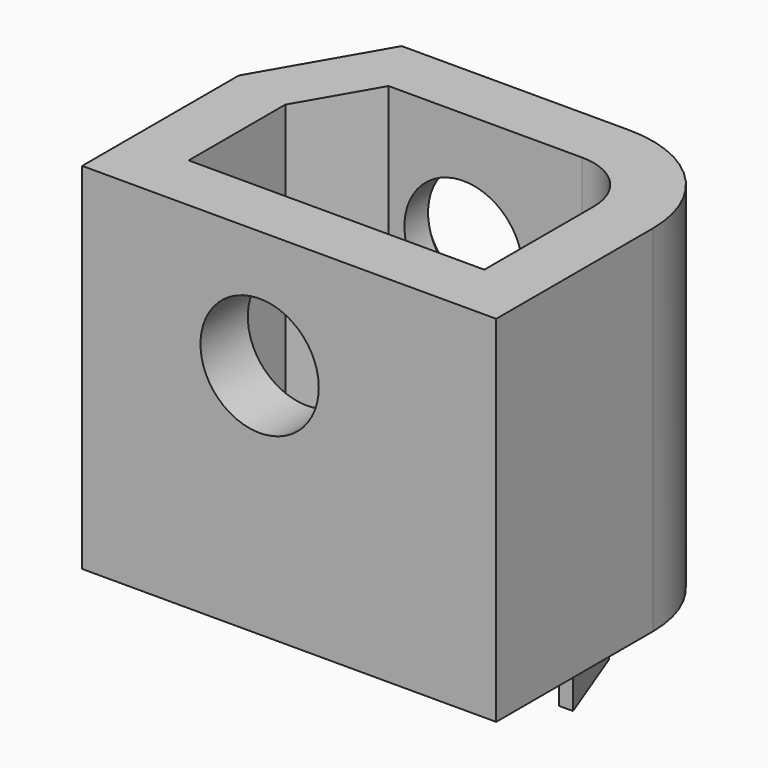
from build123d import *

# Parameters (mm, degrees)
F1_DEPTH       = 6
F2_SIZE2       = 1.1547005384
F2_SIZE        = 2
F3_T           = -1
F4_TEXT_SIZE   = 2.7020308254
F5_DEPTH       = 1
F7_D           = 2
F7_CSINK_D     = 3
F7_CSINK_ANGLE = 90


# Not quite as in the source:
# - Text() gives the source's letters only with a copy of the font that has no kerning and outlines rounded to 1/6400 em; it was checked with that copy


with BuildPart() as f1:
    # F0 (on Top) → F1 (new body)
    with BuildSketch(Plane.XY):
        with BuildLine():
            Line((1.5, 5.31), (-3.5, 5.31))
            Line((-3.5, 5.31), (-3.5, 0))
            Line((-3.5, 0), (3.5, 0))
            Line((3.5, 0), (3.5, 3.31))
            ThreePointArc((3.5, 3.31), (2.9142135624, 4.7242135624), (1.5, 5.31))
        make_face()
    extrude(amount=F1_DEPTH)

    # F2
    f2_edges = [f1.edges().sort_by_distance(p)[0] for p in [
        (-3.5, 5.31, 3),
    ]]
    f2_side = f1.faces().sort_by_distance((-3.5, 2.655, 3))[0]
    chamfer(f2_edges, length=F2_SIZE, length2=F2_SIZE2, reference=f2_side)

    # F3
    f3_openings = [f1.faces().sort_by_distance(p)[0] for p in [
        (0.027763, 2.535777, 6),
    ]]
    offset(amount=F3_T, openings=f3_openings)

    # F4 (on face) → F5 (join)
    with BuildSketch(Plane(origin=(0, 0, 0), x_dir=(1, 0, 0), z_dir=(0, 0, -1))):
        with Locations((0, -3.8215573877)):
            Text('2v', F4_TEXT_SIZE, font='Open Sans', text_align=(TextAlign.LEFT, TextAlign.BOTTOM))
    extrude(amount=F5_DEPTH)

    # F7 (through all)
    with Locations(Plane(origin=(0, 5.31, 0), x_dir=(-1, 0, 0), z_dir=(0, 1, 0))):
        with Locations((0.5, 4)):
            CounterSinkHole(F7_D / 2, F7_CSINK_D / 2, counter_sink_angle=F7_CSINK_ANGLE)


solid = f1.part
